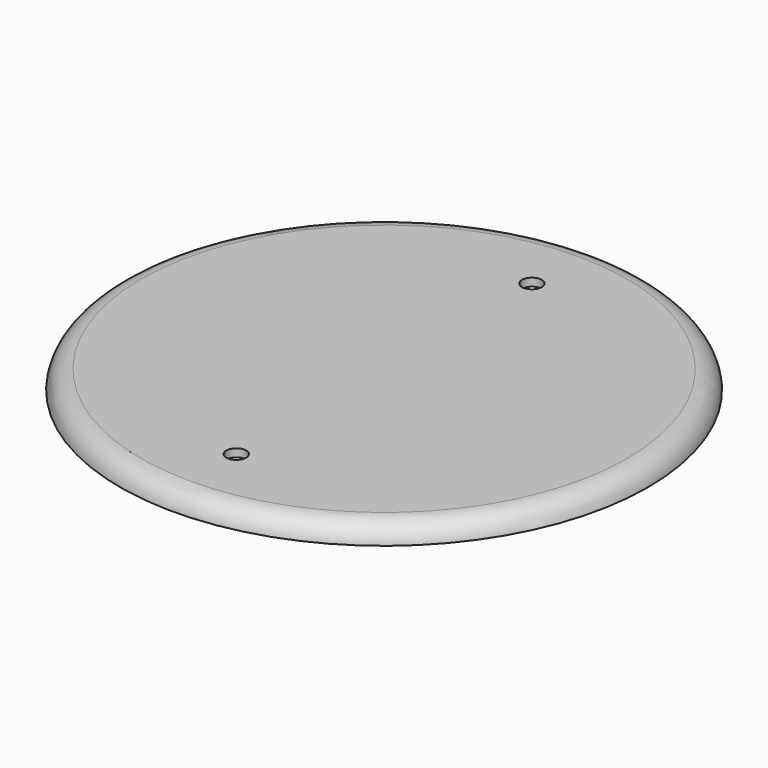
from build123d import *

# Parameters (mm, degrees)
F0_R     = 63.5
F1_DEPTH = 1.905
F2_R     = 2.38125
F3_DEPTH = 1.906
F4_R     = 63.5
F4_R_2   = 60.96
F5_DEPTH = 2.54


# Not quite as in the source:
# - a fillet or chamfer that OpenCascade refuses, or shapes differently, is made with other operations: its cross-section is extruded or revolved along the edge and cut away or added


with BuildPart() as f1:
    # F0 (on Top) → F1 (new body)
    with BuildSketch(Plane.XY):
        Circle(F0_R)
    extrude(amount=F1_DEPTH)

    # F2 (on face) → F3 (cut, through all)
    with BuildSketch(Plane.XY.offset(1.905)):
        with Locations((0, 44.45)):
            Circle(F2_R)
        with Locations((0, -44.45)):
            Circle(F2_R)
    extrude(amount=-F3_DEPTH, mode=Mode.SUBTRACT)

    # F4 (on face) → F5 (join)
    with BuildSketch(Plane(origin=(0, 0, 0), x_dir=(1, 0, 0), z_dir=(0, 0, -1))):
        Circle(F4_R)
        Circle(F4_R_2, mode=Mode.SUBTRACT)
    extrude(amount=F5_DEPTH)

    # F6: fillet of radius 5.08 on 1 edges, made by hand

    # F6_s1 → F6_t2 (revolve, cut)
    with BuildSketch(Plane.XZ):
        with BuildLine():
            ThreePointArc((63.5, -2.54), (61.8199479175, 0.635), (58.4598437524, 1.905))
            Line((58.4598437524, 1.905), (63.5, 1.905))
            Line((63.5, 1.905), (63.5, -2.54))
        make_face()
    revolve(axis=Axis((0, 0, 1.905), (0, 0, 1)), mode=Mode.SUBTRACT)


solid = f1.part
